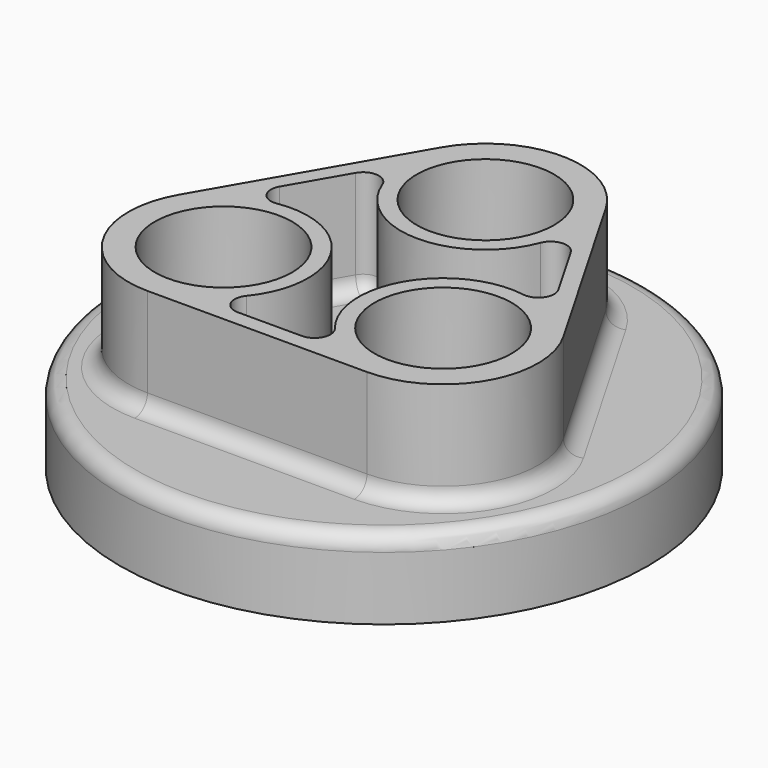
from build123d import *

# Parameters (mm, degrees)
F1_R     = 50
F1_R_2   = 16
F1_R_3   = 13
F2_DEPTH = 15
F3_T     = -3
F0_R     = 13
F4_DEPTH = 20
F5_DEPTH = 15.001
F6_DEPTH = 15
F7_R     = 3


with BuildPart() as f2:
    # F1 (on Top) → F2 (new body)
    with BuildSketch(Plane.XY):
        Circle(F1_R)
        with Locations((-20.7846096908, -12)):
            Circle(F1_R_2, mode=Mode.SUBTRACT)
        with Locations((20.7846096908, -12)):
            Circle(F1_R_2, mode=Mode.SUBTRACT)
        with Locations((0, 24)):
            Circle(F1_R_2, mode=Mode.SUBTRACT)
        with Locations((-20.7846096908, -12)):
            Circle(F1_R_2)
        with Locations((-20.7846096908, -12)):
            Circle(F1_R_3, mode=Mode.SUBTRACT)
        with Locations((-20.7846096908, -12)):
            Circle(F1_R_3)
        with Locations((0, 24)):
            Circle(F1_R_2)
        with Locations((0, 24)):
            Circle(F1_R_3, mode=Mode.SUBTRACT)
        with Locations((0, 24)):
            Circle(F1_R_3)
        with Locations((20.7846096908, -12)):
            Circle(F1_R_2)
        with Locations((20.7846096908, -12)):
            Circle(F1_R_3, mode=Mode.SUBTRACT)
        with Locations((20.7846096908, -12)):
            Circle(F1_R_3)
    extrude(amount=-F2_DEPTH)

    # F3
    f3_openings = [f2.faces().sort_by_distance(p)[0] for p in [
        (0, 0, -15),
    ]]
    offset(amount=F3_T, openings=f3_openings)

    # F0 (on Top) → F4 (join)
    with BuildSketch(Plane.XY):
        with BuildLine():
            ThreePointArc((15.5884572681, 33), (0, 42), (-15.5884572681, 33))
            Line((-15.5884572681, 33), (-36.3730669589, -3))
            ThreePointArc((-36.3730669589, -3), (-36.3730669589, -21), (-20.7846096908, -30))
            Line((-20.7846096908, -30), (20.7846096908, -30))
            ThreePointArc((20.7846096908, -30), (36.3730669589, -21), (36.3730669589, -3))
            Line((36.3730669589, -3), (15.5884572681, 33))
        make_face()
        with Locations((-20.7846096908, -12)):
            Circle(F0_R, mode=Mode.SUBTRACT)
        with BuildLine():
            ThreePointArc((-20.3558409881, 18.7426491778), (-17.5180367181, 20.2330555813), (-14.9539071804, 18.3095993076))
            ThreePointArc((-14.9539071804, 18.3095993076), (0, 8), (14.9539071804, 18.3095993076))
            ThreePointArc((14.9539071804, 18.3095993076), (17.5180367181, 20.2330555813), (20.3558409881, 18.7426491778))
            Line((20.3558409881, 18.7426491778), (26.4095308163, 8.2573508222))
            ThreePointArc((26.4095308163, 8.2573508222), (26.2813584886, 5.0545370316), (23.3335317237, 3.7956638503))
            ThreePointArc((23.3335317237, 3.7956638503), (6.9282032303, -4), (8.3796245433, -22.1052631579))
            ThreePointArc((8.3796245433, -22.1052631579), (8.7633217705, -25.2875926129), (6.0536898282, -27))
            Line((6.0536898282, -27), (-6.0536898282, -27))
            ThreePointArc((-6.0536898282, -27), (-8.7633217705, -25.2875926129), (-8.3796245433, -22.1052631579))
            ThreePointArc((-8.3796245433, -22.1052631579), (-6.9282032303, -4), (-23.3335317237, 3.7956638503))
            ThreePointArc((-23.3335317237, 3.7956638503), (-26.2813584886, 5.0545370316), (-26.4095308163, 8.2573508222))
            Line((-26.4095308163, 8.2573508222), (-20.3558409881, 18.7426491778))
        make_face(mode=Mode.SUBTRACT)
        with Locations((20.7846096908, -12)):
            Circle(F0_R, mode=Mode.SUBTRACT)
        with Locations((0, 24)):
            Circle(F0_R, mode=Mode.SUBTRACT)
    extrude(amount=F4_DEPTH)

    # F0 (on Top) → F5 (cut, through all)
    with BuildSketch(Plane.XY):
        with Locations((0, 24)):
            Circle(F0_R)
        with Locations((-20.7846096908, -12)):
            Circle(F0_R)
        with Locations((20.7846096908, -12)):
            Circle(F0_R)
    extrude(amount=-F5_DEPTH, mode=Mode.SUBTRACT)

    # F1 (on Top) → F6 (join, through all)
    with BuildSketch(Plane.XY):
        with Locations((0, 24)):
            Circle(F1_R_2)
        with Locations((0, 24)):
            Circle(F1_R_3, mode=Mode.SUBTRACT)
        with Locations((20.7846096908, -12)):
            Circle(F1_R_2)
        with Locations((20.7846096908, -12)):
            Circle(F1_R_3, mode=Mode.SUBTRACT)
        with Locations((-20.7846096908, -12)):
            Circle(F1_R_2)
        with Locations((-20.7846096908, -12)):
            Circle(F1_R_3, mode=Mode.SUBTRACT)
    extrude(amount=-F6_DEPTH)

    # F7
    f7_edges = [f2.edges().sort_by_distance(p)[0] for p in [
        (23.382686, 13.5, 0),
        (0, -30, 0),
        (-50, 0, 0),
        (-47, 0, -3),
        (-36.78461, -12, -3),
        (4.78461, -12, -3),
        (-16, 24, -3),
        (-26.281358, 5.054537, 0),
        (-23.382686, 13.5, 0),
        (-6.928203, -4, 0),
        (-8.763322, -25.287593, 0),
        (0, -27, 0),
        (8.763322, -25.287593, 0),
        (6.928203, -4, 0),
        (26.281358, 5.054537, 0),
        (17.518037, 20.233056, 0),
        (0, 8, 0),
        (-17.518037, 20.233056, 0),
        (25.980762, 15, 0),
        (36.373067, -21, 0),
        (-36.373067, -21, 0),
        (-25.980762, 15, 0),
        (0, 42, 0),
    ]]
    fillet(f7_edges, radius=F7_R)


solid = f2.part
